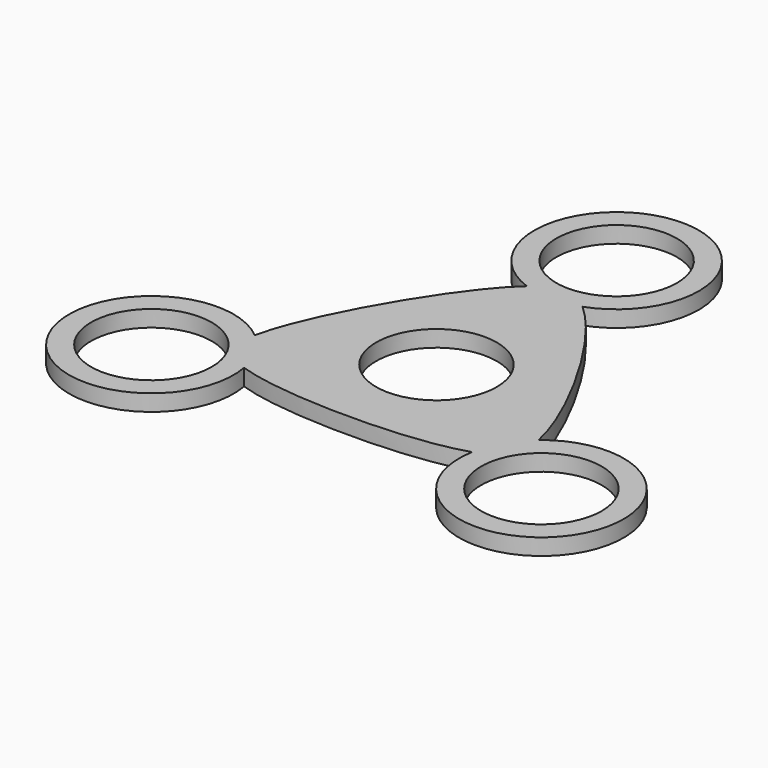
from build123d import *

# Parameters (mm, degrees)
F0_R     = 11
F1_DEPTH = 3


with BuildPart() as f1:
    # F0 (on Top) → F1 (new body)
    with BuildSketch(Plane.XY):
        with BuildLine():
            add(Edge.make_bspline(
                [(5.0692520794, 26.9407597389), (1.3719432198, 30.1629827921), (-1.3719432198, 30.1629827921), (-5.0692520794, 26.9407597389)],
                knots=[0.8898242879, 0.8898242879, 0.8898242879, 0.8898242879, 1, 1, 1, 1], degree=3))
            ThreePointArc((5.0692520794, 26.9407597389), (0, 56.0582199693), (-5.0692520794, 26.9407597389))
        make_face()
        with Locations((0, 41.0582199693)):
            Circle(F0_R, mode=Mode.SUBTRACT)
        with BuildLine():
            add(Edge.make_bspline(
                [(25.8660083708, -9.0802787905), (23.9582735086, 0.6684610246), (12.5580409831, 20.414242977), (5.0692520794, 26.9407597389)],
                knots=[0.6666666667, 0.6666666667, 0.6666666667, 0.6666666667, 0.8898242879, 0.8898242879, 0.8898242879, 0.8898242879], degree=3))
            add(Edge.make_bspline(
                [(5.0692520794, 26.9407597389), (1.3719432198, 30.1629827921), (-1.3719432198, 30.1629827921), (-5.0692520794, 26.9407597389)],
                knots=[0.8898242879, 0.8898242879, 0.8898242879, 0.8898242879, 1, 1, 1, 1], degree=3))
            add(Edge.make_bspline(
                [(-5.0692520794, 26.9407597389), (-12.5580409831, 20.414242977), (-23.9582735086, 0.6684610246), (-25.8660083708, -9.0802787905)],
                knots=[0, 0, 0, 0, 0.2231576212, 0.2231576212, 0.2231576212, 0.2231576212], degree=3))
            add(Edge.make_bspline(
                [(-25.8660083708, -9.0802787905), (-26.8078809618, -13.8933537152), (-25.435937742, -16.2696290769), (-20.7967562915, -17.8604809484)],
                knots=[0.2231576212, 0.2231576212, 0.2231576212, 0.2231576212, 0.3333333333, 0.3333333333, 0.3333333333, 0.3333333333], degree=3))
            add(Edge.make_bspline(
                [(-20.7967562915, -17.8604809484), (-11.4002325256, -21.0827040016), (11.4002325256, -21.0827040016), (20.7967562915, -17.8604809484)],
                knots=[0.3333333333, 0.3333333333, 0.3333333333, 0.3333333333, 0.5564909546, 0.5564909546, 0.5564909546, 0.5564909546], degree=3))
            add(Edge.make_bspline(
                [(20.7967562915, -17.8604809484), (25.435937742, -16.2696290769), (26.8078809618, -13.8933537152), (25.8660083708, -9.0802787905)],
                knots=[0.5564909546, 0.5564909546, 0.5564909546, 0.5564909546, 0.6666666667, 0.6666666667, 0.6666666667, 0.6666666667], degree=3))
        make_face()
        Circle(F0_R, mode=Mode.SUBTRACT)
        with BuildLine():
            ThreePointArc((20.7967562915, -17.8604809484), (48.5478425843, -28.0291099846), (25.8660083708, -9.0802787905))
            add(Edge.make_bspline(
                [(20.7967562915, -17.8604809484), (25.435937742, -16.2696290769), (26.8078809618, -13.8933537152), (25.8660083708, -9.0802787905)],
                knots=[0.5564909546, 0.5564909546, 0.5564909546, 0.5564909546, 0.6666666667, 0.6666666667, 0.6666666667, 0.6666666667], degree=3))
        make_face()
        with Locations((35.5574615276, -20.5291099846)):
            Circle(F0_R, mode=Mode.SUBTRACT)
        with BuildLine():
            add(Edge.make_bspline(
                [(-25.8660083708, -9.0802787905), (-26.8078809618, -13.8933537152), (-25.435937742, -16.2696290769), (-20.7967562915, -17.8604809484)],
                knots=[0.2231576212, 0.2231576212, 0.2231576212, 0.2231576212, 0.3333333333, 0.3333333333, 0.3333333333, 0.3333333333], degree=3))
            ThreePointArc((-25.8660083708, -9.0802787905), (-48.5478425843, -28.0291099846), (-20.7967562915, -17.8604809484))
        make_face()
        with Locations((-35.5574615276, -20.5291099846)):
            Circle(F0_R, mode=Mode.SUBTRACT)
    extrude(amount=F1_DEPTH)


solid = f1.part
